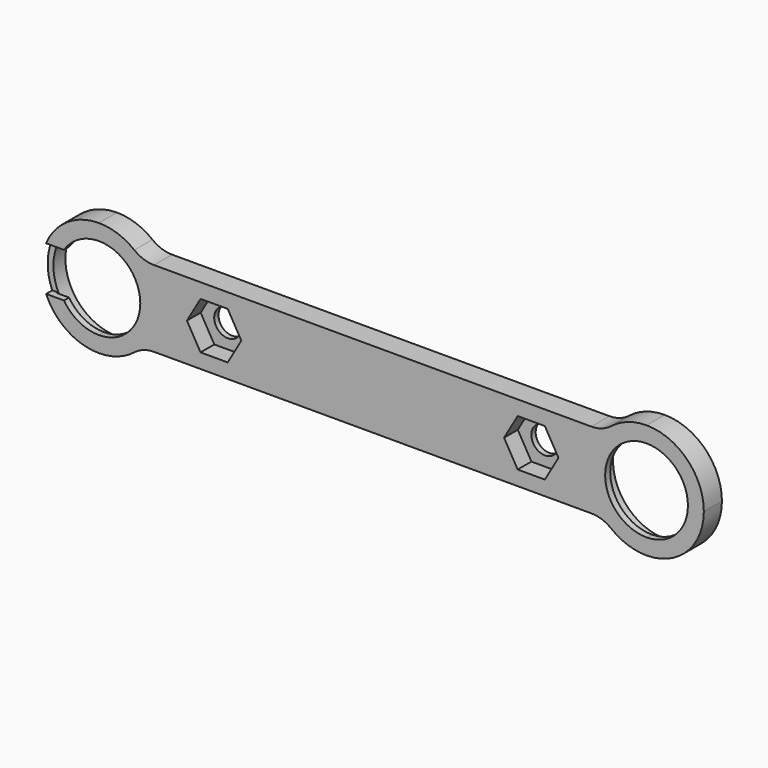
from build123d import *

# Parameters (mm, degrees)
F1_DEPTH = 3.55
F2_R     = 8.1
F3_DEPTH = 2.55
F4_R     = 5
F5_R     = 2.15
F6_DEPTH = 2.7
F7_DEPTH = 3.551
F8_W     = 1.2
F8_H     = 7
F9_DEPTH = 200


# Not quite as in the source:
# - a feature names something its author has since deleted; it is built from what else it names


with BuildPart() as f1:
    # F0 (on Front) → F1 (new body)
    with BuildSketch(Plane.XZ):
        with BuildLine():
            Line((0, 6.5), (0, 9))
            ThreePointArc((0, 9), (-9, 0), (0, -9))
            Line((0, -9), (0, -6.5))
            ThreePointArc((0, -6.5), (-6.5, 0), (0, 6.5))
        make_face()
        with BuildLine():
            ThreePointArc((6.7082039325, -6), (8.4075512307, -3.211398808), (9, 0))
            ThreePointArc((9, 0), (8.4075512307, 3.211398808), (6.7082039325, 6))
            ThreePointArc((6.7082039325, 6), (3.6742346142, 8.2158383626), (0, 9))
            Line((0, 9), (0, 6.5))
            ThreePointArc((0, 6.5), (4.5961940777, 4.5961940777), (6.5, 0))
            ThreePointArc((6.5, 0), (4.5961940777, -4.5961940777), (0, -6.5))
            Line((0, -6.5), (0, -9))
            ThreePointArc((0, -9), (3.6742346142, -8.2158383626), (6.7082039325, -6))
        make_face()
        with BuildLine():
            ThreePointArc((86, 9), (82.3257653858, 8.2158383626), (79.2917960675, 6))
            ThreePointArc((79.2917960675, 6), (77, 0), (79.2917960675, -6))
            ThreePointArc((79.2917960675, -6), (82.3257653858, -8.2158383626), (86, -9))
            Line((86, -9), (86, -6.5))
            ThreePointArc((86, -6.5), (79.5, 0), (86, 6.5))
            Line((86, 6.5), (86, 9))
        make_face()
        with BuildLine():
            ThreePointArc((95, 0), (92.3639610307, 6.3639610307), (86, 9))
            Line((86, 9), (86, 6.5))
            ThreePointArc((86, 6.5), (90.5961940777, 4.5961940777), (92.5, 0))
            ThreePointArc((92.5, 0), (90.5961940777, -4.5961940777), (86, -6.5))
            Line((86, -6.5), (86, -9))
            ThreePointArc((86, -9), (92.3639610307, -6.3639610307), (95, 0))
        make_face()
        with BuildLine():
            ThreePointArc((6.7082039325, 6), (8.4075512307, 3.211398808), (9, 0))
            ThreePointArc((9, 0), (8.4075512307, -3.211398808), (6.7082039325, -6))
            Line((6.7082039325, -6), (79.2917960675, -6))
            ThreePointArc((79.2917960675, -6), (77, 0), (79.2917960675, 6))
            Line((79.2917960675, 6), (6.7082039325, 6))
        make_face()
    extrude(amount=F1_DEPTH)

    # F2 (on face) → F3 (cut)
    with BuildSketch(Plane.XZ):
        Circle(F2_R)
        with Locations((86, 0)):
            Circle(F2_R)
    extrude(amount=F3_DEPTH, mode=Mode.SUBTRACT)

    # F4
    f4_edges = [f1.edges().sort_by_distance(p)[0] for p in [
        (6.708204, -1.775, -6),
        (6.708204, -1.775, 6),
        (79.291796, -1.775, 6),
        (79.291796, -1.775, -6),
    ]]
    fillet(f4_edges, radius=F4_R)

    # F5 (on face) → F6 (cut)
    with BuildSketch(Plane.XZ.offset(3.55)):
        Polygon((22.372391992, 0), (20.236195996, 3.7), (15.963804004, 3.7), (13.827608008, 0), (15.963804004, -3.7), (20.236195996, -3.7), align=None)
        with Locations((18.1, 0)):
            Circle(F5_R, mode=Mode.SUBTRACT)
        Polygon((63.627608008, 0), (65.763804004, -3.7), (70.036195996, -3.7), (72.172391992, 0), (70.036195996, 3.7), (65.763804004, 3.7), align=None)
        with Locations((67.9, 0)):
            Circle(F5_R, mode=Mode.SUBTRACT)
    extrude(amount=-F6_DEPTH, mode=Mode.SUBTRACT)

    # F5 (on face) → F7 (cut, through all)
    with BuildSketch(Plane.XZ.offset(3.55)):
        with Locations((18.1, 0)):
            Circle(F5_R)
        with Locations((67.9, 0)):
            Circle(F5_R)
    extrude(amount=-F7_DEPTH, mode=Mode.SUBTRACT)

    # F8 (on Right) → F9 (cut)
    with BuildSketch(Plane.YZ):
        with Locations((-2.95, 0)):
            Rectangle(F8_W, F8_H)
    extrude(amount=-F9_DEPTH, mode=Mode.SUBTRACT)


solid = f1.part
